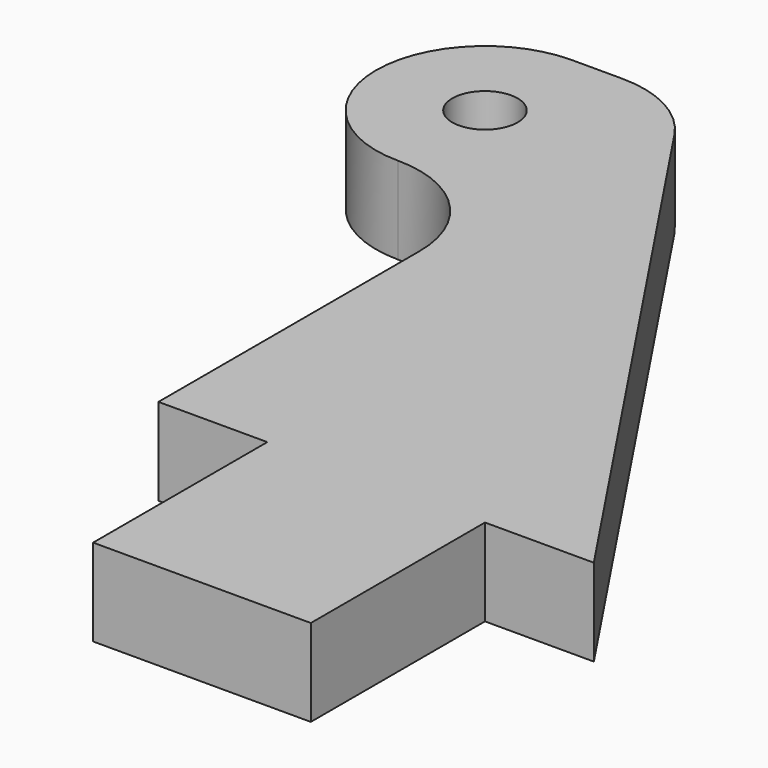
from build123d import *

# Parameters (mm, degrees)
F0_R     = 0.75
F0_W     = 5
F0_H     = 5
F1_DEPTH = 2
F2_R     = 2.49999


# Not quite as in the source:
# - a fillet or chamfer is up to 0.001 mm smaller than in the source, because OpenCascade refuses the exact size


with BuildPart() as f1:
    # F0 (on Top) → F1 (new body)
    with BuildSketch(Plane.XY):
        Polygon((-5, 0), (-2.5, 0), (2.5, 0), (5, 0), (-5, 15), (-10, 15), (-10, 10), (-5, 10), align=None)
        with Locations((-7.5, 12.5)):
            Circle(F0_R, mode=Mode.SUBTRACT)
        with Locations((0, -2.5)):
            Rectangle(F0_W, F0_H)
    extrude(amount=F1_DEPTH)

    # F2 (radius 2.5 in the source; OpenCascade refuses exactly that, so slightly less here)
    f2_edges = [f1.edges().sort_by_distance(p)[0] for p in [
        (-10, 15, 1),
        (-10, 10, 1),
        (-5, 15, 1),
        (-5, 10, 1),
    ]]
    fillet(f2_edges, radius=F2_R)


solid = f1.part
